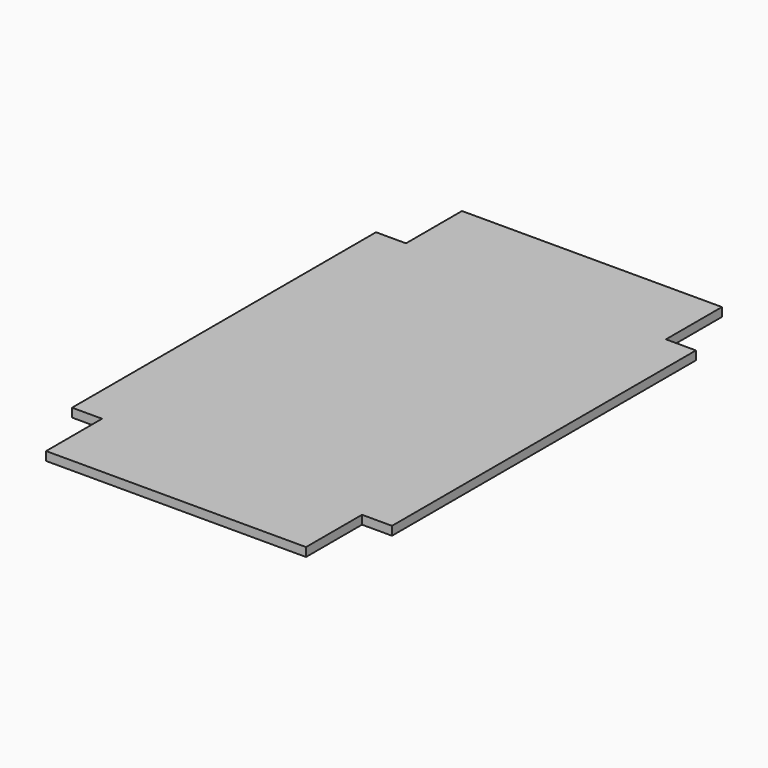
from build123d import *

# Parameters (mm, degrees)
F0_W             = 406.4
F0_H             = 660.4
F1_DEPTH         = 11.1125
F2_W             = 38.1
F2_H             = 88.9
F3_DEPTH         = 25.4
F3_COPIES2_COUNT = 2


# Not quite as in the source:
# - a pattern or mirror of a feature is missing from the dataset's text; its kind, count and spacing are read off the source's solid


with BuildPart() as f1:
    # F0 (on Top) → F1 (new body)
    with BuildSketch(Plane.XY):
        Rectangle(F0_W, F0_H)
    extrude(amount=F1_DEPTH)

    # F2 (on face) → F3 (cut)
    with BuildSketch(Plane.XY.offset(11.1125)):
        with Locations((-184.15, -285.75)):
            Rectangle(F2_W, F2_H)
    f3 = extrude(amount=-F3_DEPTH, mode=Mode.SUBTRACT)

    # F3_copies: F3 across plane
    add(f3.mirror(Plane(origin=(0, 0, 0), x_dir=(0, 0, 1), z_dir=(1, 0, 0))), mode=Mode.SUBTRACT)

    # F3_copies1: F3 across plane
    add(f3.mirror(Plane.ZX), mode=Mode.SUBTRACT)

    # F3_copies2: F3 ×2 about axis
    f3_copies2_axis = Axis((0, 0, 0), (0, 0, 1))
    for i in range(1, F3_COPIES2_COUNT):
        add(f3.rotate(f3_copies2_axis, i * 360 / F3_COPIES2_COUNT), mode=Mode.SUBTRACT)


solid = f1.part
